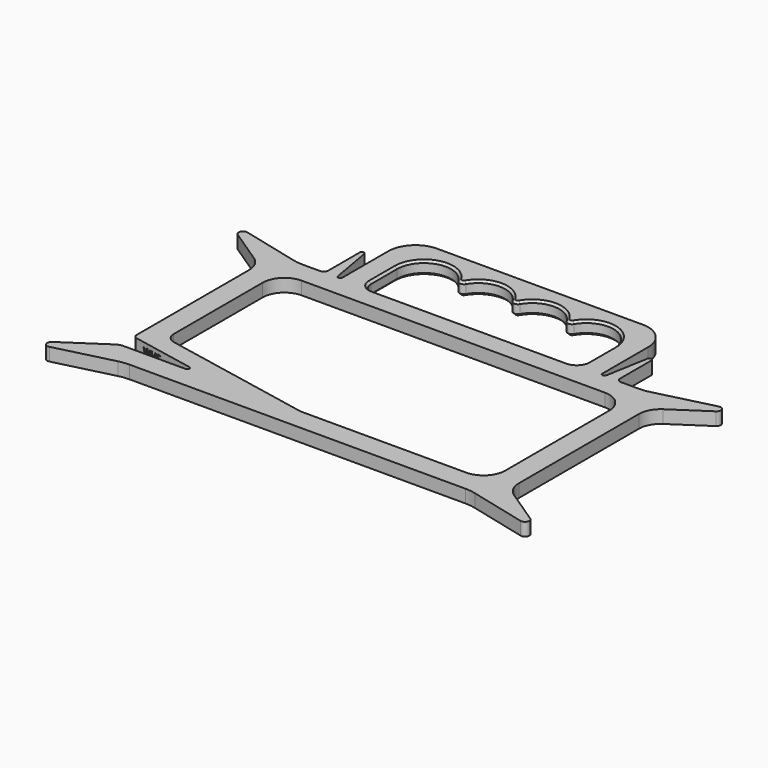
from build123d import *

# Parameters (mm, degrees)
F1_DEPTH     = 6
F2_SIZE      = 1
F3_SIZE      = 1
F4_TEXT_SIZE = 4.4435301485
F5_DEPTH     = 1


# Not quite as in the source:
# - a feature names something its author has since deleted; it is built from what else it names
# - Text() gives the source's letters only with a copy of the font that has no kerning and outlines rounded to 1/6400 em; it was checked with that copy


with BuildPart() as f1:
    # F0 (on Top) → F1 (new body)
    with BuildSketch(Plane.XY):
        with BuildLine():
            ThreePointArc((-82.3885999884, -50.5971499971), (-79.9815527616, -50.1498488663), (-77.5378874876, -50))
            Line((-77.5378874876, -50), (77.5378874876, -50))
            ThreePointArc((77.5378874876, -50), (79.9815527616, -50.1498488663), (82.3885999884, -50.5971499971))
            Line((82.3885999884, -50.5971499971), (108.7983199584, -57.1995799896))
            ThreePointArc((108.7983199584, -57.1995799896), (111.1124197999, -56.068402159), (110.392791601, -53.5951944006))
            Line((110.392791601, -53.5951944006), (94.4529980377, -42.9686653585))
            ThreePointArc((94.4529980377, -42.9686653585), (91.1832540123, -39.3667416704), (90, -34.6481624151))
            Line((90, -34.6481624151), (90, 34.6481624151))
            ThreePointArc((90, 34.6481624151), (91.1832540123, 39.3667416704), (94.4529980377, 42.9686653585))
            Line((94.4529980377, 42.9686653585), (110.392791601, 53.5951944006))
            ThreePointArc((110.392791601, 53.5951944006), (111.1124197999, 56.068402159), (108.7983199584, 57.1995799896))
            Line((108.7983199584, 57.1995799896), (82.3885999884, 50.5971499971))
            ThreePointArc((82.3885999884, 50.5971499971), (79.9815527616, 50.1498488663), (77.5378874876, 50))
            Line((77.5378874876, 50), (69.4173235893, 50))
            ThreePointArc((69.4173235893, 50), (68.003110027, 50.5857864376), (67.4173235893, 52))
            Line((67.4173235893, 52), (67.4173235893, 70.2056278168))
            ThreePointArc((67.4173235893, 70.2056278168), (66.5044793321, 71.2018225149), (65.4325158363, 70.3792759945))
            Line((65.4325158363, 70.3792759945), (61.984807753, 50.8263518223))
            ThreePointArc((61.984807753, 50.8263518223), (60.9128442573, 50.0038053019), (60, 51))
            Line((60, 51), (60, 77.5))
            ThreePointArc((60, 77.5), (56.3388347648, 86.3388347648), (47.5, 90))
            Line((47.5, 90), (-47.5, 90))
            ThreePointArc((-47.5, 90), (-56.3388347648, 86.3388347648), (-60, 77.5))
            Line((-60, 77.5), (-60, 51))
            ThreePointArc((-60, 51), (-60.9128442573, 50.0038053019), (-61.984807753, 50.8263518223))
            Line((-61.984807753, 50.8263518223), (-65.4325158363, 70.3792759945))
            ThreePointArc((-65.4325158363, 70.3792759945), (-66.5044793321, 71.2018225149), (-67.4173235893, 70.2056278168))
            Line((-67.4173235893, 70.2056278168), (-67.4173235893, 52))
            ThreePointArc((-67.4173235893, 52), (-68.003110027, 50.5857864376), (-69.4173235893, 50))
            Line((-69.4173235893, 50), (-77.5378874876, 50))
            ThreePointArc((-77.5378874876, 50), (-79.9815527616, 50.1498488663), (-82.3885999884, 50.5971499971))
            Line((-82.3885999884, 50.5971499971), (-108.7983199584, 57.1995799896))
            ThreePointArc((-108.7983199584, 57.1995799896), (-111.1124197999, 56.068402159), (-110.392791601, 53.5951944006))
            Line((-110.392791601, 53.5951944006), (-94.4529980377, 42.9686653585))
            ThreePointArc((-94.4529980377, 42.9686653585), (-91.1832540123, 39.3667416704), (-90, 34.6481624151))
            Line((-90, 34.6481624151), (-90, -30.3378421815))
            ThreePointArc((-90, -30.3378421815), (-89.5450183526, -31.6078493823), (-88.3870817099, -32.3000266147))
            Line((-88.3870817099, -32.3000266147), (-59.3970795566, -38.0189077834))
            ThreePointArc((-59.3970795566, -38.0189077834), (-58.5953585826, -39.0972311252), (-59.5906204116, -40))
            Line((-59.5906204116, -40), (-68.7849670649, -40))
            Line((-68.7849670649, -40), (-70.7849670649, -40))
            Line((-70.7849670649, -40), (-80, -40))
            Line((-80, -40), (-88.4861218113, -40))
            ThreePointArc((-88.4861218113, -40), (-89.9350425548, -40.2145398676), (-91.2596227925, -40.8397485283))
            Line((-91.2596227925, -40.8397485283), (-110.392791601, -53.5951944006))
            ThreePointArc((-110.392791601, -53.5951944006), (-111.1124197999, -56.068402159), (-108.7983199584, -57.1995799896))
            Line((-108.7983199584, -57.1995799896), (-82.3885999884, -50.5971499971))
        make_face()
        with BuildLine():
            Line((-70, 40), (70, 40))
            ThreePointArc((70, 40), (77.0710678119, 37.0710678119), (80, 30))
            Line((80, 30), (80, -30))
            ThreePointArc((80, -30), (77.0710678119, -37.0710678119), (70, -40))
            Line((70, -40), (-6.0610717578, -40))
            ThreePointArc((-6.0610717578, -40), (-6.5472273837, -39.9763091451), (-7.0287760326, -39.905461083))
            Line((-7.0287760326, -39.905461083), (-75.9677042748, -26.3058229584))
            ThreePointArc((-75.9677042748, -26.3058229584), (-78.8625458816, -24.5753798774), (-80, -21.4003618754))
            Line((-80, -21.4003618754), (-80, 30))
            ThreePointArc((-80, 30), (-77.0710678119, 37.0710678119), (-70, 40))
        make_face(mode=Mode.SUBTRACT)
        with BuildLine():
            ThreePointArc((50, 55), (48.5355339059, 51.4644660941), (45, 50))
            Line((45, 50), (-45, 50))
            ThreePointArc((-45, 50), (-48.5355339059, 51.4644660941), (-50, 55))
            Line((-50, 55), (-50, 70))
            ThreePointArc((-50, 70), (-40.7826608215, 82.0612660169), (-26.724137931, 76.3348872658))
            ThreePointArc((-26.724137931, 76.3348872658), (-25, 75.3484692283), (-23.275862069, 76.3348872658))
            ThreePointArc((-23.275862069, 76.3348872658), (-12.5, 82.5), (-1.724137931, 76.3348872658))
            ThreePointArc((-1.724137931, 76.3348872658), (0, 75.3484692283), (1.724137931, 76.3348872658))
            ThreePointArc((1.724137931, 76.3348872658), (12.5, 82.5), (23.275862069, 76.3348872658))
            ThreePointArc((23.275862069, 76.3348872658), (25, 75.3484692283), (26.724137931, 76.3348872658))
            ThreePointArc((26.724137931, 76.3348872658), (40.7826608215, 82.0612660169), (50, 70))
            Line((50, 70), (50, 55))
        make_face(mode=Mode.SUBTRACT)
    extrude(amount=F1_DEPTH)

    # F2
    f2_edges = [f1.edges().sort_by_distance(p)[0] for p in [
        (-50, 62.5, 6),
        (-40.782661, 82.061266, 6),
        (-25, 75.348469, 6),
    ]]
    chamfer(f2_edges, length=F2_SIZE)

    # F3
    f3_edges = [f1.edges().sort_by_distance(p)[0] for p in [
        (40.782661, 82.061266, 0),
        (25, 75.348469, 0),
        (50, 62.5, 0),
        (0, 50, 0),
        (48.535534, 51.464466, 0),
    ]]
    chamfer(f3_edges, length=F3_SIZE)

    # F4 (on face) → F5 (cut)
    with BuildSketch(Plane(origin=(-9.4439839609, -47.8731953482, 0), x_dir=(0.9810922166, -0.193540855, 0), z_dir=(-0.193540855, -0.9810922166, 0))):
        with Locations((-76.7387151718, 0.9068096988)):
            Text('WHS', F4_TEXT_SIZE, font='Open Sans', text_align=(TextAlign.LEFT, TextAlign.BOTTOM))
    extrude(amount=-F5_DEPTH, mode=Mode.SUBTRACT)


solid = f1.part
